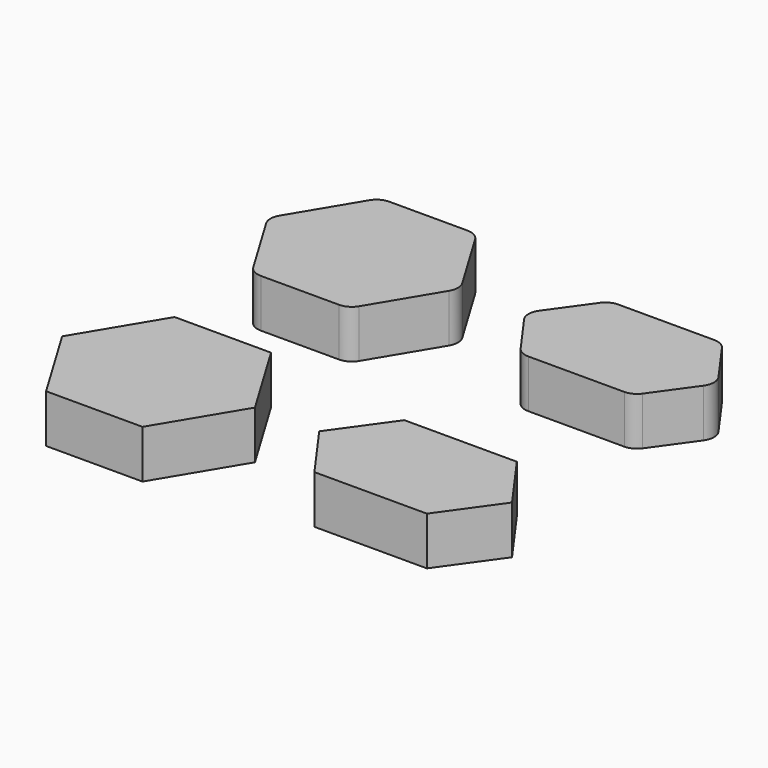
from build123d import *

# Parameters (mm, degrees)
F1_DEPTH = 9.525
F2_R     = 3.175
F2_2_R   = 3.175


# Not quite as in the source:
# - a feature names something its author has since deleted; it is built from what else it names


with BuildPart() as f1:
    # F0 (on Top) → F1 (new body)
    with BuildSketch(Plane.XY):
        Polygon((-19.05, 50.8), (-9.525, 34.925), (9.525, 34.925), (19.05, 50.8), (9.525, 66.675), (-9.525, 66.675), align=None)
    extrude(amount=-F1_DEPTH)

    # F2
    f2_edges = [f1.edges().sort_by_distance(p)[0] for p in [
        (-19.05, 50.8, -4.7625),
        (-9.525, 34.925, -4.7625),
        (19.05, 50.8, -4.7625),
        (9.525, 34.925, -4.7625),
        (9.525, 66.675, -4.7625),
        (-9.525, 66.675, -4.7625),
    ]]
    fillet(f2_edges, radius=F2_R)


with BuildPart() as f1b:
    # F0 (on Top) → F1, piece 2 (new body)
    with BuildSketch(Plane.XY):
        Polygon((31.7499993861, 50.8), (39.6874993861, 39.6875), (61.9124993861, 39.6875), (69.8499993861, 50.8), (61.9124993861, 61.9125), (39.6874993861, 61.9125), align=None)
    extrude(amount=-F1_DEPTH)

    # F2#2
    f2_2_edges = [f1b.edges().sort_by_distance(p)[0] for p in [
        (31.749999, 50.8, -4.7625),
        (39.687499, 61.9125, -4.7625),
        (61.912499, 61.9125, -4.7625),
        (69.849999, 50.8, -4.7625),
        (61.912499, 39.6875, -4.7625),
        (39.687499, 39.6875, -4.7625),
    ]]
    fillet(f2_2_edges, radius=F2_2_R)


with BuildPart() as f1c:
    # F0 (on Top) → F1, piece 3 (new body)
    with BuildSketch(Plane.XY):
        Polygon((-19.05, 0), (-9.525, -15.875), (9.525, -15.875), (19.05, 0), (9.525, 15.875), (-9.525, 15.875), align=None)
    extrude(amount=-F1_DEPTH)


with BuildPart() as f1d:
    # F0 (on Top) → F1, piece 4 (new body)
    with BuildSketch(Plane.XY):
        Polygon((31.7499993861, 0), (39.6874993861, -11.1125), (61.9124993861, -11.1125), (69.8499993861, 0), (61.9124993861, 11.1125), (39.6874993861, 11.1125), align=None)
    extrude(amount=-F1_DEPTH)


solid = Compound([f1.part, f1b.part, f1c.part, f1d.part])
